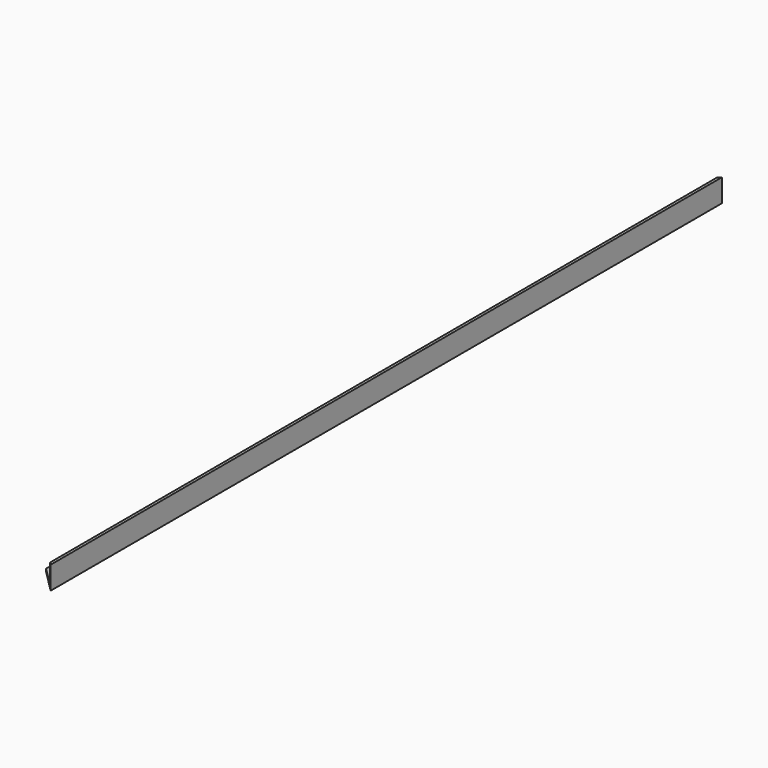
from build123d import *

# Parameters (mm, degrees)
F1_DEPTH    = 920
F2_T1_DEPTH = 47.7168298797
F4_DEPTH    = 25
F5_T1_DEPTH = 47.7168298797
F7_DEPTH    = 25


# Not quite as in the source:
# - a fillet or chamfer that OpenCascade refuses, or shapes differently, is made with other operations: its cross-section is extruded or revolved along the edge and cut away or added


with BuildPart() as f1:
    # F0 (on Front) → F1 (new body)
    with BuildSketch(Plane.XZ):
        Polygon((0, 3), (0, 0), (25, 0), (25, 25), (22, 25), (22, 3), align=None)
    extrude(amount=F1_DEPTH)

    # F2: chamfer of 5 on 1 edges, made by hand

    # F2_s2 → F2_t1 (cut)
    with BuildSketch(Plane.XY.offset(-9.8584149398)):
        Polygon((22, -5), (27, 0), (22, 0), align=None)
    extrude(amount=F2_T1_DEPTH, mode=Mode.SUBTRACT)

    # F3 (on face) → F4 (cut)
    with BuildSketch(Plane.XY.offset(3)):
        Polygon((0, -27), (22, -5), (22, 0), (0, 0), align=None)
    extrude(amount=-F4_DEPTH, mode=Mode.SUBTRACT)

    # F5: chamfer of 5 on 1 edges, made by hand

    # F5_s2 → F5_t1 (cut)
    with BuildSketch(Plane.XY.offset(-9.8584149398)):
        Polygon((22, -915), (27, -920), (22, -920), align=None)
    extrude(amount=F5_T1_DEPTH, mode=Mode.SUBTRACT)

    # F6 (on face) → F7 (cut)
    with BuildSketch(Plane.XY.offset(3)):
        Polygon((22, -920), (22, -915), (0, -893), (0, -920), align=None)
    extrude(amount=-F7_DEPTH, mode=Mode.SUBTRACT)


solid = f1.part
